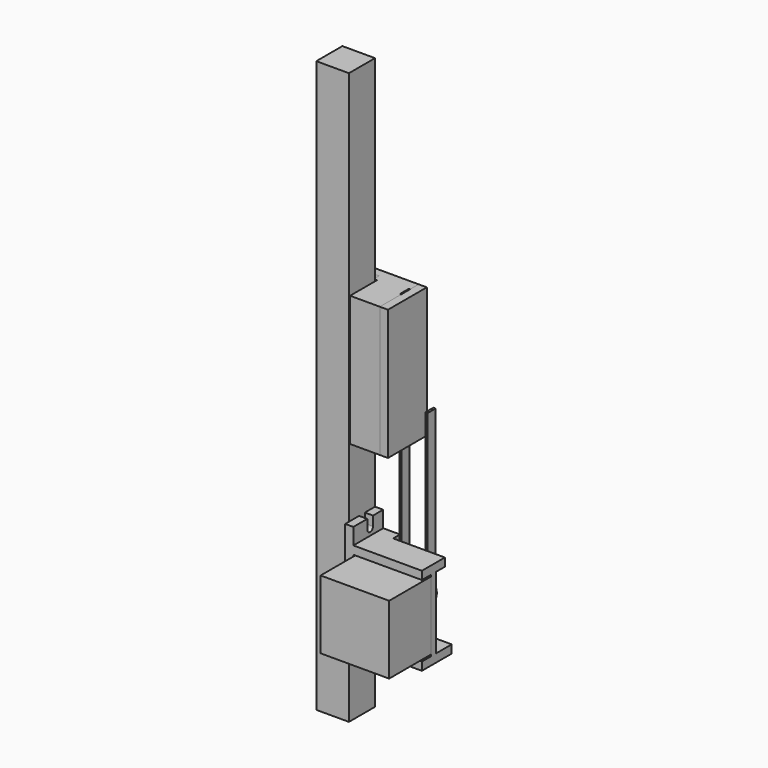
from build123d import *

# Parameters (mm, degrees)
F1_W           = 20
F1_H           = 20
F2_DEPTH       = 300
F2_DEPTH_BACK  = 50
F3_W           = 42
F3_H           = 32
F4_DEPTH       = 42
F5_R           = 2.5
F6_DEPTH       = 20
F7_R           = 8.65
F8_DEPTH       = 14.3
F9_R           = 1.5
F10_DEPTH      = 4
F11_R          = 2.75
F12_DEPTH      = 3
F14_DEPTH      = 43
F14_DEPTH_BACK = 1
F16_DEPTH      = 5
F17_W          = 22.85
F17_H          = 5
F18_DEPTH      = 42
F19_W          = 31.65
F19_H          = 5.25
F20_DEPTH      = 5
F22_W          = 17
F22_H          = 5
F23_DEPTH      = 80
F24_R          = 1.05
F25_DEPTH      = 5
F27_R          = 8.65
F27_R_2        = 7.27
F28_DEPTH      = 3.6
F28_DEPTH_BACK = 3.6
F30_DEPTH      = 3
F30_DEPTH_BACK = 3
F32_DEPTH      = 80
F33_R          = 1.65
F34_DEPTH      = 5
F36_W          = 29.75
F36_H          = 80
F37_DEPTH      = 5


# Not quite as in the source:
# - a feature names something its author has since deleted; it is built from what else it names


with BuildPart() as f2:
    # F1 (on Top) → F2 (new body, two sides)
    with BuildSketch(Plane.XY) as f2_sk:
        Rectangle(F1_W, F1_H)
    extrude(amount=F2_DEPTH)
    extrude(f2_sk.sketch, amount=-F2_DEPTH_BACK)


with BuildPart() as f4:
    # F3 (on Top) → F4 (new body)
    with BuildSketch(Plane.XY):
        with Locations((36, -21.95)):
            Rectangle(F3_W, F3_H)
    extrude(amount=F4_DEPTH)

    # F5 (on face) → F6 (join)
    with BuildSketch(Plane(origin=(0, -5.95, 0), x_dir=(-1, 0, 0), z_dir=(0, 1, 0))):
        with Locations((-36, 21)):
            Circle(F5_R)
    extrude(amount=F6_DEPTH)

    # F7 (on face) → F8 (join)
    with BuildSketch(Plane(origin=(0, 14.05, 0), x_dir=(-1, 0, 0), z_dir=(0, 1, 0))):
        with Locations((-36, 21)):
            Circle(F7_R)
    extrude(amount=-F8_DEPTH)

    # F9 (on face) → F10 (join)
    with BuildSketch(Plane(origin=(0, -5.95, 0), x_dir=(-1, 0, 0), z_dir=(0, 1, 0))):
        with Locations((-51.5, 36.5)):
            Circle(F9_R)
        with Locations((-51.5, 5.5)):
            Circle(F9_R)
        with Locations((-20.5, 36.5)):
            Circle(F9_R)
        with Locations((-20.5, 5.5)):
            Circle(F9_R)
    extrude(amount=F10_DEPTH)

    # F11 (on face) → F12 (join)
    with BuildSketch(Plane(origin=(0, -1.95, 0), x_dir=(-1, 0, 0), z_dir=(0, 1, 0))):
        with Locations((-20.5, 36.5)):
            Circle(F11_R)
        with Locations((-20.5, 5.5)):
            Circle(F11_R)
        with Locations((-51.5, 36.5)):
            Circle(F11_R)
        with Locations((-51.5, 5.5)):
            Circle(F11_R)
    extrude(amount=F12_DEPTH)

    # F27 (on offset) → F28 (cut, two sides)
    with BuildSketch(Plane(origin=(0, 10.05, 0), x_dir=(-1, 0, 0), z_dir=(0, 1, 0))) as f28_sk:
        with Locations((-36, 21)):
            Circle(F27_R)
        with Locations((-36, 21)):
            Circle(F27_R_2, mode=Mode.SUBTRACT)
    extrude(amount=F28_DEPTH, mode=Mode.SUBTRACT)
    extrude(f28_sk.sketch, amount=-F28_DEPTH_BACK, mode=Mode.SUBTRACT)


with BuildPart() as f14:
    # F13 (on Top) → F14 (new body, two sides)
    with BuildSketch(Plane.XY) as f14_sk:
        Polygon((57, -1.95), (15, -1.95), (15, 4.05), (15, 10), (10, 10), (10, -12.85), (15, -12.85), (15, -5.95), (57, -5.95), align=None)
    extrude(amount=F14_DEPTH)
    extrude(f14_sk.sketch, amount=-F14_DEPTH_BACK)

    # F15 (on face) → F16 (join, through all)
    with BuildSketch(Plane(origin=(10, 0, 0), x_dir=(0, -1, 0), z_dir=(-1, 0, 0))):
        with BuildLine():
            Line((-10, 43), (12.85, 43))
            Line((12.85, 43), (12.85, 58))
            Line((12.85, 58), (2.2, 58))
            Line((2.2, 58), (2.2, 52.2))
            ThreePointArc((2.2, 52.2), (0, 50), (-2.2, 52.2))
            Line((-2.2, 52.2), (-2.2, 58))
            Line((-2.2, 58), (-10, 58))
            Line((-10, 58), (-10, 43))
        make_face()
        with BuildLine():
            Line((-2.2, -16), (-2.2, -10.2))
            ThreePointArc((-2.2, -10.2), (0, -8), (2.2, -10.2))
            Line((2.2, -10.2), (2.2, -16))
            Line((2.2, -16), (12.85, -16))
            Line((12.85, -16), (12.85, -1))
            Line((12.85, -1), (-10, -1))
            Line((-10, -1), (-10, -16))
            Line((-10, -16), (-2.2, -16))
        make_face()
    extrude(amount=-F16_DEPTH)

    # F17 (on face) → F18 (join, through all)
    with BuildSketch(Plane.YZ.offset(15)):
        with Locations((-1.425, 45.5)):
            Rectangle(F17_W, F17_H)
        with Locations((-1.425, -3.5)):
            Rectangle(F17_W, F17_H)
    extrude(amount=F18_DEPTH)

    # F19 (on face) → F20 (cut, through all)
    with BuildSketch(Plane.XY.offset(48)):
        with Locations((41.175, 7.375)):
            Rectangle(F19_W, F19_H)
    extrude(amount=-F20_DEPTH, mode=Mode.SUBTRACT)


with BuildPart() as f23:
    # F22 (on offset) → F23 (new body)
    with BuildSketch(Plane.XY.offset(100)):
        with Locations((0, 12.5)):
            Rectangle(F22_W, F22_H)
    extrude(amount=F23_DEPTH)

    # F24 (on face) → F25 (cut, through all)
    with BuildSketch(Plane(origin=(0, 15, 0), x_dir=(-1, 0, 0), z_dir=(0, 1, 0))):
        with Locations((0, 165)):
            Circle(F24_R)
        with Locations((0, 140)):
            Circle(F24_R)
        with Locations((0, 115)):
            Circle(F24_R)
    extrude(amount=-F25_DEPTH, mode=Mode.SUBTRACT)


with BuildPart() as f30:
    # F29 (on offset) → F30 (new body, two sides)
    with BuildSketch(Plane(origin=(0, 10.05, 0), x_dir=(-1, 0, 0), z_dir=(0, 1, 0))) as f30_sk:
        with BuildLine():
            Line((-44.65, 121), (-44.65, 21))
            ThreePointArc((-44.65, 21), (-36, 12.35), (-27.35, 21))
            Line((-27.35, 21), (-27.35, 121))
            Line((-27.35, 121), (-28.73, 121))
            Line((-28.73, 121), (-28.73, 21))
            ThreePointArc((-28.73, 21), (-36, 13.73), (-43.27, 21))
            Line((-43.27, 21), (-43.27, 121))
            Line((-43.27, 121), (-44.65, 121))
        make_face()
    extrude(amount=F30_DEPTH)
    extrude(f30_sk.sketch, amount=-F30_DEPTH_BACK)


with BuildPart() as f32:
    # F31 (on offset) → F32 (new body)
    with BuildSketch(Plane.XY.offset(100)):
        Polygon((-8.5, 20), (-8.5, 15), (8.5, 15), (8.5, 11), (10.5, 11), (10.5, -9.75), (28.73, -9.75), (28.73, 6.55), (27.98, 6.55), (27.98, 13.55), (28.73, 13.55), (28.73, 20), align=None)
    extrude(amount=F32_DEPTH)

    # F33 (on face) → F34 (cut, through all)
    with BuildSketch(Plane(origin=(0, 20, 0), x_dir=(-1, 0, 0), z_dir=(0, 1, 0))):
        with Locations((0, 165)):
            Circle(F33_R)
        with Locations((0, 140)):
            Circle(F33_R)
        with Locations((0, 115)):
            Circle(F33_R)
    extrude(amount=-F34_DEPTH, mode=Mode.SUBTRACT)


with BuildPart() as f37:
    # F36 (on offset) → F37 (new body)
    with BuildSketch(Plane.YZ.offset(28.73)):
        with Locations((5.125, 140)):
            Rectangle(F36_W, F36_H)
    extrude(amount=F37_DEPTH)


solid = Compound([f2.part, f4.part, f14.part, f23.part, f30.part, f32.part, f37.part])
